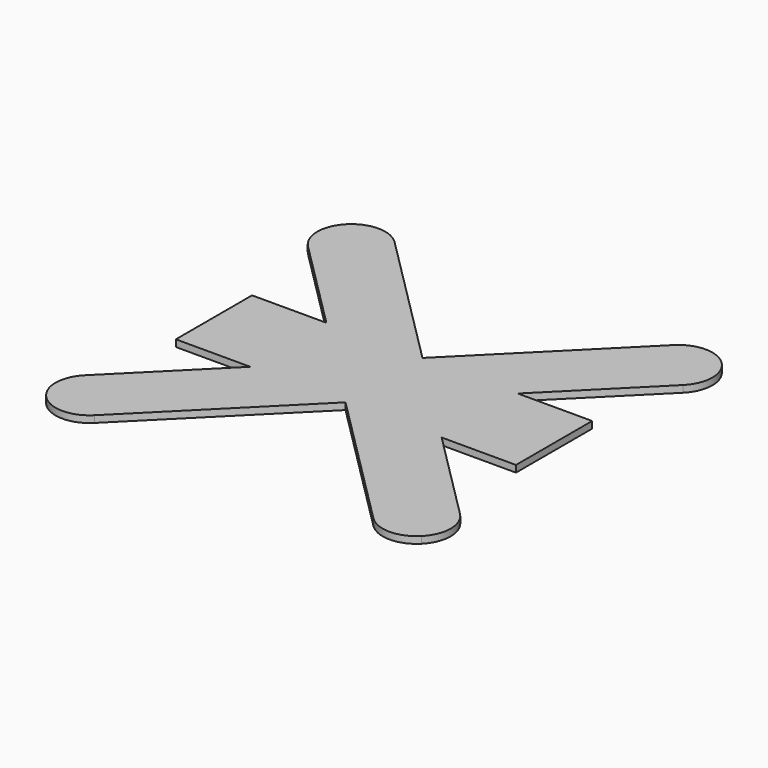
from build123d import *

# Parameters (mm, degrees)
F1_W     = 10
F1_H     = 34
F1_H_2   = 10
F1_W_2   = 34
F2_DEPTH = 1
F3_ANGLE = 45
F4_W     = 50
F4_H     = 14
F5_DEPTH = 1
F6_R     = 4.99999


# Not quite as in the source:
# - a fillet or chamfer is up to 0.001 mm smaller than in the source, because OpenCascade refuses the exact size


with BuildPart() as f2:
    # F1 (on Top) → F2 (new body)
    with BuildSketch(Plane.XY):
        with Locations((0, -22)):
            Rectangle(F1_W, F1_H)
        Rectangle(F1_W, F1_H_2)
        with Locations((22, 0)):
            Rectangle(F1_W_2, F1_H_2)
        with Locations((-22, 0)):
            Rectangle(F1_W_2, F1_H_2)
        with Locations((0, 22)):
            Rectangle(F1_W, F1_H)
    extrude(amount=F2_DEPTH)


with BuildPart() as f2_1:
    # F3: moved
    add(f2.part.rotate(Axis((0, 0, 15.9228555858), (0, 0, 1)), F3_ANGLE))

    # F4 (on Top) → F5 (join)
    with BuildSketch(Plane.XY):
        Rectangle(F4_W, F4_H)
    extrude(amount=F5_DEPTH)

    # F6 (radius 5 in the source; OpenCascade refuses exactly that, so slightly less here)
    f6_edges = [f2_1.edges().sort_by_distance(p)[0] for p in [
        (-31.112698, 24.041631, 0.5),
        (-31.112698, -24.041631, 0.5),
        (-24.041631, -31.112698, 0.5),
        (24.041631, -31.112698, 0.5),
        (31.112698, 24.041631, 0.5),
        (31.112698, -24.041631, 0.5),
        (24.041631, 31.112698, 0.5),
        (-24.041631, 31.112698, 0.5),
    ]]
    fillet(f6_edges, radius=F6_R)


solid = f2_1.part
